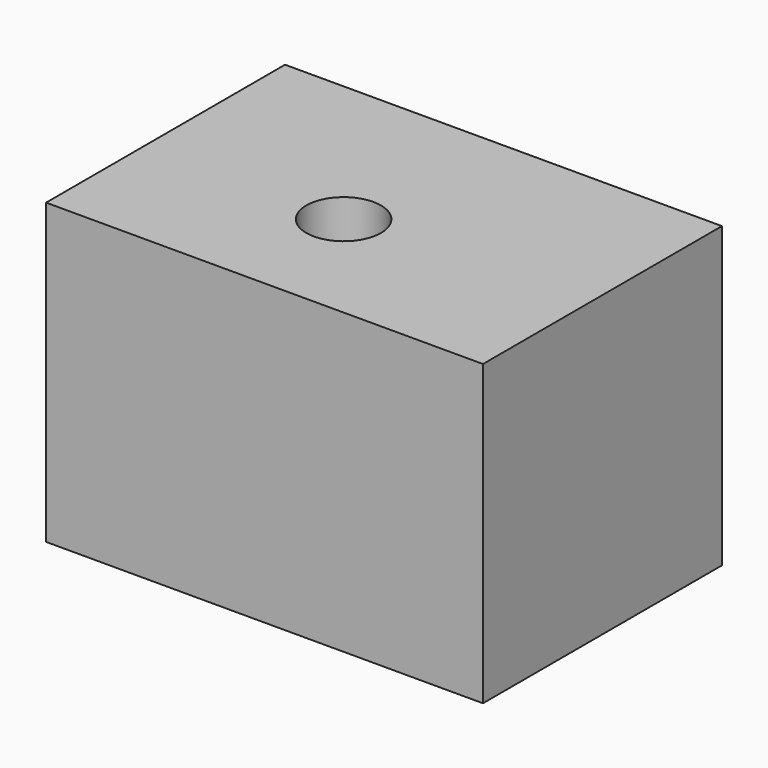
from build123d import *

# Parameters (mm, degrees)
F0_W     = 74.3044822258
F0_H     = 50.8
F1_DEPTH = 50.8
F5_D     = 12.7
F7_DEPTH = 12.7


# Not quite as in the source:
# - the program builds the solid bodies; features that only make, move or delete a surface that nothing else refers to are left out


with BuildPart() as f1:
    # F0 (on Front) → F1 (new body)
    with BuildSketch(Plane.XZ):
        with Locations((-44.8397286236, 28.155177366)):
            Rectangle(F0_W, F0_H)
    extrude(amount=F1_DEPTH)

    # F5 (through all)
    with Locations(Plane.XY.offset(53.555177366)):
        with Locations((-48.1568910182, -29.835857451)):
            Hole(F5_D / 2)


with BuildPart() as f7:
    # F6 (on face) → F7 (new body)
    with BuildSketch(Plane.XZ):
        Polygon((-40.3997157671, 32.0204286902), (-45.6071044348, 37.2297600777), (-52.9728378235, 37.231133788), (-58.182169211, 32.0237451204), (-58.1835429214, 24.6580117316), (-52.9761542537, 19.4486803441), (-45.6104208649, 19.4473066338), (-40.4010894774, 24.6546953015), align=None)
    extrude(amount=-F7_DEPTH)


solid = Compound([f1.part, f7.part])
